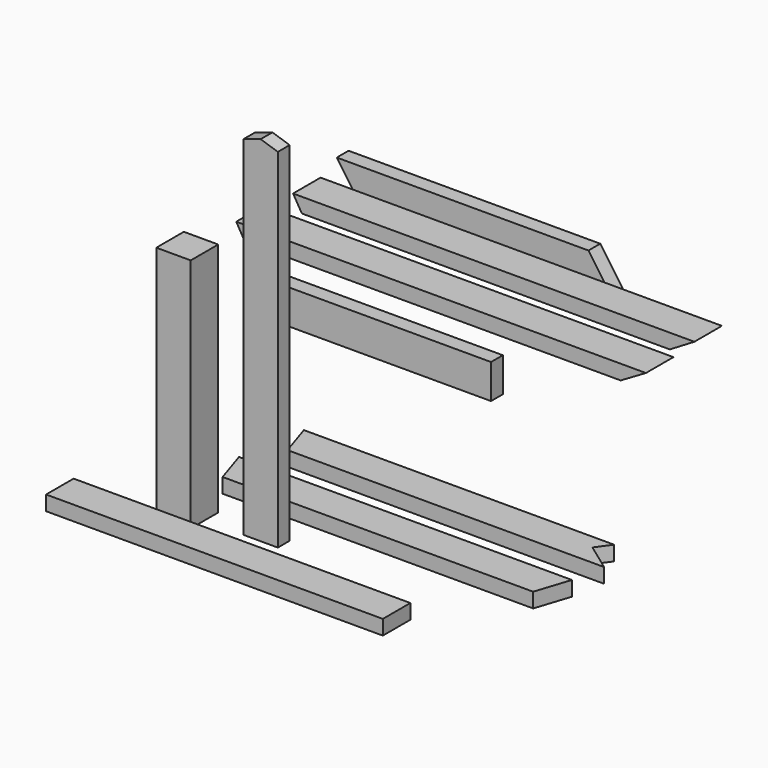
from build123d import *

# Parameters (mm, degrees)
F0_W      = 88.9
F0_H      = 88.9
F1_DEPTH  = 609.6
F2_W      = 88.9
F2_H      = 38.1
F3_DEPTH  = 914.4
F5_DEPTH  = 44.451
F6_W      = 88.9
F6_H      = 38.1
F7_DEPTH  = 802.386
F9_DEPTH  = 38.1
F10_W     = 88.9
F10_H     = 38.1
F11_DEPTH = 1058.418
F13_DEPTH = 88.901
F15_DEPTH = 291.4930525193
F16_W     = 88.9
F16_H     = 38.1
F17_DEPTH = 869.95
F18_W     = 88.9
F18_H     = 38.1
F19_DEPTH = 1036.828
F21_DEPTH = 886.4102444897
F22_DEPTH = 886.4102444897
F23_W     = 88.9
F23_H     = 38.1
F24_DEPTH = 1066.8
F26_DEPTH = 38.101
F28_DEPTH = 38.101
F29_W     = 38.1
F29_H     = 88.9
F30_DEPTH = 558.8
F31_W     = 38.1
F31_H     = 88.9
F32_DEPTH = 762
F34_DEPTH = 976.812467675
F36_DEPTH = 976.812467675
F37_W     = 88.9
F37_H     = 38.1
F38_DEPTH = 508
F40_DEPTH = 38.101
F42_DEPTH = 38.101


with BuildPart() as f1:
    # F0 (on Top) → F1 (new body)
    with BuildSketch(Plane.XY):
        Rectangle(F0_W, F0_H)
    extrude(amount=F1_DEPTH)


with BuildPart() as f3:
    # F2 (on Top) → F3 (new body)
    with BuildSketch(Plane.XY):
        with Locations((189.5409819244, 19.05)):
            Rectangle(F2_W, F2_H)
    extrude(amount=F3_DEPTH)

    # F4 (on face) → F5 (cut, through all)
    with BuildSketch(Plane.XZ):
        Polygon((145.0909819244, 899.9573195024), (189.5409819244, 914.4), (145.0909819244, 914.4), align=None)
        Polygon((233.9909819244, 914.4), (189.5409819244, 914.4), (233.9909819244, 899.9573195024), align=None)
    extrude(amount=-F5_DEPTH, mode=Mode.SUBTRACT)


with BuildPart() as f7:
    # F6 (on Right) → F7 (new body)
    with BuildSketch(Plane.YZ):
        with Locations((158.5839751139, 19.05)):
            Rectangle(F6_W, F6_H)
    extrude(amount=F7_DEPTH)

    # F8 (on face) → F9 (join)
    with BuildSketch(Plane.XY.offset(38.1)):
        Polygon((-28.8853609951, 203.0339751139), (0, 114.1339751139), (0, 203.0339751139), align=None)
        Polygon((802.386, 203.0339751139), (802.386, 114.1339751139), (831.2713609951, 203.0339751139), align=None)
    extrude(amount=-F9_DEPTH)


with BuildPart() as f11:
    # F10 (on Right) → F11 (new body)
    with BuildSketch(Plane.YZ):
        with Locations((202.5920525193, 581.7884122946)):
            Rectangle(F10_W, F10_H)
    extrude(amount=F11_DEPTH)

    # F12 (on face) → F13 (cut, through all)
    with BuildSketch(Plane.XZ.offset(-158.1420525193)):
        Polygon((1058.418, 562.7384122946), (1058.418, 600.8384122946), (993.0868510167, 562.7384122946), align=None)
    extrude(amount=-F13_DEPTH, mode=Mode.SUBTRACT)

    # F14 (on face) → F15 (cut, through all)
    with BuildSketch(Plane(origin=(0, 247.0420525193, 0), x_dir=(-1, 0, 0), z_dir=(0, 1, 0))):
        Polygon((0, 562.7384122946), (0, 600.8384122946), (-22.2192632854, 562.7384122946), align=None)
    extrude(amount=-F15_DEPTH, mode=Mode.SUBTRACT)


with BuildPart() as f17:
    # F16 (on Right) → F17 (new body)
    with BuildSketch(Plane.YZ):
        with Locations((-411.4587221622, 210.9255347661)):
            Rectangle(F16_W, F16_H)
    extrude(amount=F17_DEPTH)


with BuildPart() as f19:
    # F18 (on Right) → F19 (new body)
    with BuildSketch(Plane.YZ):
        with Locations((386.0505223274, 571.2980129524)):
            Rectangle(F18_W, F18_H)
    extrude(amount=F19_DEPTH)

    # F20 (on face) → F21 (cut, through all)
    with BuildSketch(Plane(origin=(0, 430.5005223274, 0), x_dir=(-1, 0, 0), z_dir=(0, 1, 0))):
        Polygon((0, 552.2480129524), (0, 590.3480129524), (-22.856602877, 552.2480129524), align=None)
    extrude(amount=-F21_DEPTH, mode=Mode.SUBTRACT)

    # F20 (on face) → F22 (cut, through all)
    with BuildSketch(Plane(origin=(0, 430.5005223274, 0), x_dir=(-1, 0, 0), z_dir=(0, 1, 0))):
        Polygon((-973.3185621448, 552.2480129524), (-1036.828, 590.3480129524), (-1036.828, 552.2480129524), align=None)
    extrude(amount=-F22_DEPTH, mode=Mode.SUBTRACT)


with BuildPart() as f24:
    # F23 (on Right) → F24 (new body)
    with BuildSketch(Plane.YZ):
        with Locations((332.0678491998, 19.05)):
            Rectangle(F23_W, F23_H)
    extrude(amount=F24_DEPTH)

    # F25 (on face) → F26 (cut, through all)
    with BuildSketch(Plane.XY.offset(38.1)):
        Polygon((28.8853609951, 287.6178491998), (0, 376.5178491998), (0, 287.6178491998), align=None)
    extrude(amount=-F26_DEPTH, mode=Mode.SUBTRACT)

    # F27 (on face) → F28 (cut, through all)
    with BuildSketch(Plane.XY.offset(38.1)):
        Polygon((774.8437501952, 339.8719581286), (846.7653609951, 287.6178491998), (1066.8, 287.6178491998), (1066.8, 376.5178491998), (801.4685485351, 376.5178491998), align=None)
    extrude(amount=-F28_DEPTH, mode=Mode.SUBTRACT)


with BuildPart() as f30:
    # F29 (on Right) → F30 (new body)
    with BuildSketch(Plane.YZ):
        with Locations((301.4461100101, 368.408357701)):
            Rectangle(F29_W, F29_H)
    extrude(amount=F30_DEPTH)


with BuildPart() as f32:
    # F31 (on Right) → F32 (new body)
    with BuildSketch(Plane.YZ):
        with Locations((501.8527455127, 570.2958106995)):
            Rectangle(F31_W, F31_H)
    extrude(amount=F32_DEPTH)

    # F33 (on face) → F34 (cut, through all)
    with BuildSketch(Plane(origin=(0, 520.9027455127, 0), x_dir=(-1, 0, 0), z_dir=(0, 1, 0))):
        Polygon((0, 525.8458106995), (0, 614.7458106995), (-62.2484501468, 525.8458106995), align=None)
    extrude(amount=-F34_DEPTH, mode=Mode.SUBTRACT)

    # F35 (on face) → F36 (cut, through all)
    with BuildSketch(Plane(origin=(0, 520.9027455127, 0), x_dir=(-1, 0, 0), z_dir=(0, 1, 0))):
        Polygon((-762, 525.8458106995), (-712.4884501468, 525.8458106995), (-650.24, 614.7458106995), (-762, 614.7458106995), align=None)
    extrude(amount=-F36_DEPTH, mode=Mode.SUBTRACT)


with BuildPart() as f38:
    # F37 (on face) → F38 (new body)
    with BuildSketch(Plane(origin=(110.6558194923, 35.9542552558, 0), x_dir=(0.3090169944, -0.9510565163, 0), z_dir=(-0.9510565163, -0.3090169944, 0))):
        with Locations((-1037.2092051929, 19.05)):
            Rectangle(F37_W, F37_H)
    extrude(amount=F38_DEPTH)

    # F39 (on face) → F40 (cut, through all)
    with BuildSketch(Plane.XY.offset(38.1)):
        Polygon((-630.4460123089, 839.0044752145), (-706.7319673124, 907.6926576227), (-679.2603565124, 823.1437333241), align=None)
    extrude(amount=-F40_DEPTH, mode=Mode.SUBTRACT)

    # F41 (on face) → F42 (cut, through all)
    with BuildSketch(Plane.XY.offset(38.1)):
        Polygon((-196.1236462345, 980.1243664665), (-223.5952570344, 1064.6732907652), (-244.937990438, 964.2636245761), align=None)
    extrude(amount=-F42_DEPTH, mode=Mode.SUBTRACT)


solid = Compound([f1.part, f3.part, f7.part, f11.part, f17.part, f19.part, f24.part, f30.part, f32.part])
